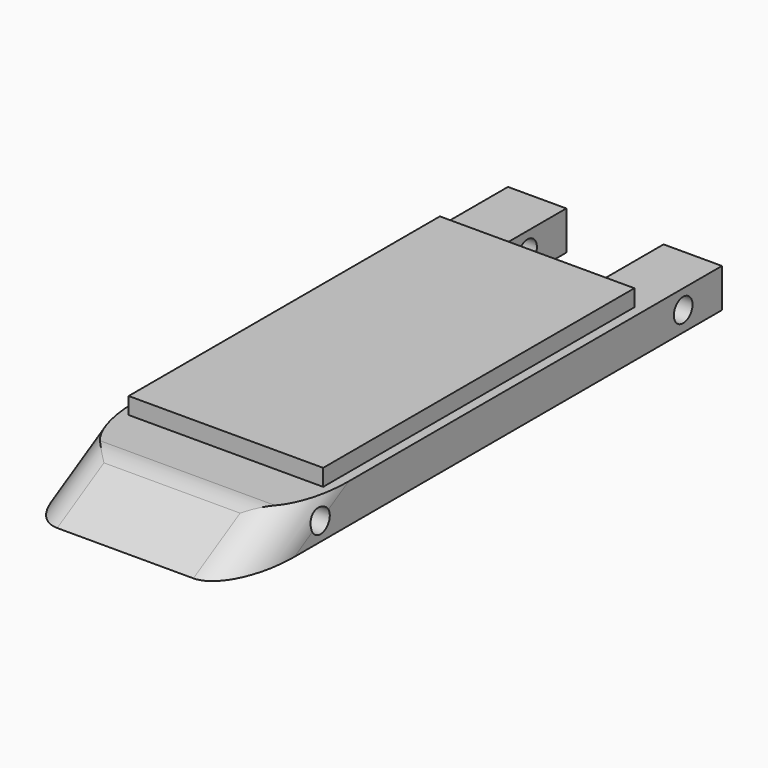
from build123d import *

# Parameters (mm, degrees)
F0_W        = 180
F0_H        = 10
F1_DEPTH    = 27.5
F2_T1_DEPTH = 261.9668603717
F3_R        = 10
F4_W        = 50
F4_H        = 100
F5_DEPTH    = 4.30577
F6_W        = 25
F6_H        = 20
F7_DEPTH    = 25
F9_D        = 6
F10_D       = 6


# Not quite as in the source:
# - a fillet or chamfer that OpenCascade refuses, or shapes differently, is made with other operations: its cross-section is extruded or revolved along the edge and cut away or added


with BuildPart() as f1:
    # F0 (on Right) → F1 (new body, symmetric)
    with BuildSketch(Plane.YZ):
        with Locations((10, -5.5927829817)):
            Rectangle(F0_W, F0_H)
    extrude(amount=F1_DEPTH, both=True)

    # F2: chamfer of 40 x 23.0940107676 on 1 edges, made by hand

    # F2_s2 → F2_t1 (cut)
    with BuildSketch(Plane.YZ.offset(-130.9834301858)):
        Polygon((-40, -0.5927829817), (-80, -23.6867937493), (-80, -0.5927829817), align=None)
    extrude(amount=F2_T1_DEPTH, mode=Mode.SUBTRACT)

    # F3
    f3_edges = [f1.edges().sort_by_distance(p)[0] for p in [
        (-27.5, -48.660254, -5.592783),
        (27.5, -48.660254, -5.592783),
        (0, -40, -0.592783),
    ]]
    fillet(f3_edges, radius=F3_R)

    # F4 (on face) → F5 (join)
    with BuildSketch(Plane.XY.offset(-0.5927829817)):
        with Locations((0, 25)):
            Rectangle(F4_W, F4_H)
    extrude(amount=F5_DEPTH)

    # F6 (on face) → F7 (cut)
    with BuildSketch(Plane.XY.offset(-0.5927829817)):
        with Locations((0, 90)):
            Rectangle(F6_W, F6_H)
    extrude(amount=-F7_DEPTH, mode=Mode.SUBTRACT)

    # F9 (through all)
    with Locations(Plane.YZ.offset(27.5)):
        with Locations((-28.9948489517, -5.8634025045)):
            Hole(F9_D / 2)

    # F10 (through all)
    with Locations(Plane.YZ.offset(27.5)):
        with Locations((87.551549077, -5.5025774054)):
            Hole(F10_D / 2)


solid = f1.part
